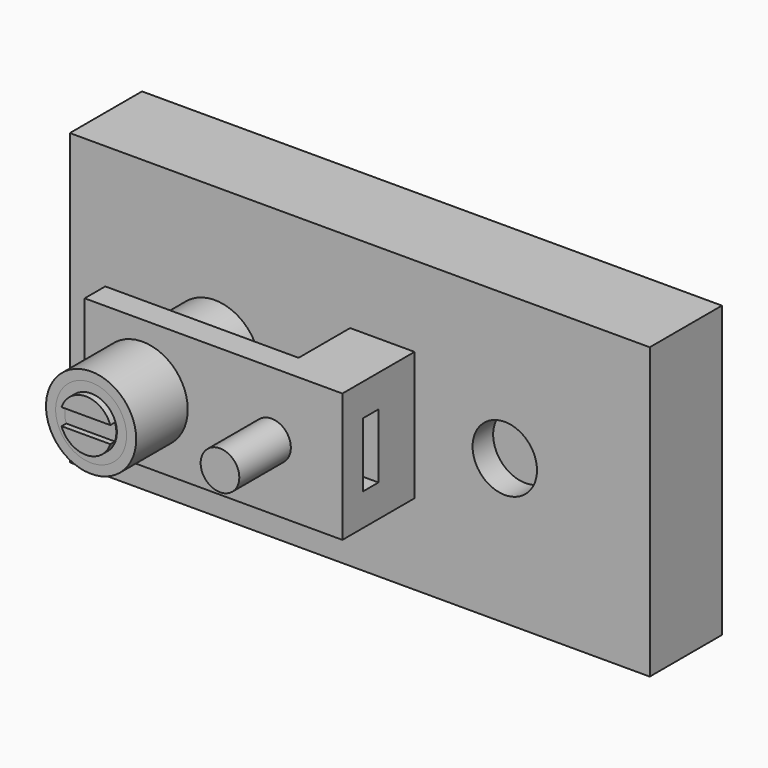
from build123d import *

# Parameters (mm, degrees)
F0_R           = 2.75
F1_DEPTH       = 7
F2_R           = 2
F3_DEPTH       = 9.9
F3_DEPTH_BACK  = 12.8
F4_R           = 3.5
F5_DEPTH       = 5
F6_R           = 2
F7_DEPTH       = 7.5
F9_START       = 7.05
F8_W           = 4
F8_H           = 1.3
F9_DEPTH       = 2
F10_W          = 20
F10_H          = 10
F11_DEPTH      = 2
F12_W          = 5
F12_H          = 5
F13_DEPTH      = 5
F14_W          = 1.5
F14_H          = 2.5
F15_DEPTH      = 22.67
F16_R          = 3.5
F16_R_2        = 2.75
F17_DEPTH      = 7
F18_R          = 2.75
F19_DEPTH      = 6.2
F19_DEPTH_BACK = 3.1
F23_START      = -5
F23_DEPTH      = 7
F25_START      = -7
F24_R          = 3.5
F25_DEPTH      = 7
F27_START      = -10
F26_W          = 32
F26_H          = 7
F27_DEPTH      = 15
F20_R          = 1.5
F28_DEPTH      = 7
F29_R          = 2.5
F30_DEPTH      = 10


with BuildPart() as f1:
    # F0 (on Front) → F1 (new body)
    with BuildSketch(Plane.XZ):
        Circle(F0_R)
    extrude(amount=F1_DEPTH)

    # F2 (on Front) → F3 (cut, two sides)
    with BuildSketch(Plane.XZ) as f3_sk:
        Circle(F2_R)
    extrude(amount=F3_DEPTH, mode=Mode.SUBTRACT)
    extrude(f3_sk.sketch, amount=-F3_DEPTH_BACK, mode=Mode.SUBTRACT)

    # F4 (on Front) → F5 (join)
    with BuildSketch(Plane.XZ):
        Circle(F4_R)
    extrude(amount=-F5_DEPTH)


with BuildPart() as f7:
    # F6 (on Front) → F7 (new body)
    with BuildSketch(Plane.XZ):
        Circle(F6_R)
    extrude(amount=F7_DEPTH)

    # F8 (on Front) → F9 (cut)
    with BuildSketch(Plane.XZ.offset(F9_START)):
        Rectangle(F8_W, F8_H)
    extrude(amount=F9_DEPTH, mode=Mode.SUBTRACT)


with BuildPart() as f11:
    # F10 (on Front) → F11 (new body)
    with BuildSketch(Plane.XZ):
        with Locations((5.5, 0)):
            Rectangle(F10_W, F10_H)
    extrude(amount=F11_DEPTH)

    # F12 (on Top) → F13 (join, symmetric)
    with BuildSketch(Plane.XY):
        with Locations((13, 2.5)):
            Rectangle(F12_W, F12_H)
    extrude(amount=F13_DEPTH, both=True)

    # F14 (on Right) → F15 (cut)
    with BuildSketch(Plane.YZ):
        with Locations((0.75, -1.25)):
            Rectangle(F14_W, F14_H)
        with Locations((0.75, 1.25)):
            Rectangle(F14_W, F14_H)
    extrude(amount=F15_DEPTH, mode=Mode.SUBTRACT)

    # F16 (on Front) → F17 (join)
    with BuildSketch(Plane.XZ):
        Circle(F16_R)
        Circle(F16_R_2, mode=Mode.SUBTRACT)
    extrude(amount=F17_DEPTH)

    # F18 (on Front) → F19 (cut, two sides)
    with BuildSketch(Plane.XZ) as f19_sk:
        Circle(F18_R)
    extrude(amount=F19_DEPTH, mode=Mode.SUBTRACT)
    extrude(f19_sk.sketch, amount=-F19_DEPTH_BACK, mode=Mode.SUBTRACT)

    # F20 (on Front) → F28 (join)
    with BuildSketch(Plane.XZ):
        with Locations((10, 0)):
            Circle(F20_R)
    extrude(amount=F28_DEPTH)


with BuildPart() as f23:
    # F22 (on Front) → F23 (new body)
    with BuildSketch(Plane.XZ.offset(F23_START)):
        Polygon((33.75, 11.25), (11.25, 11.25), (-11.25, 11.25), (-11.25, -11.25), (11.25, -11.25), (33.75, -11.25), align=None)
    extrude(amount=-F23_DEPTH)

    # F26 (on Front) → F27 (cut)
    with BuildSketch(Plane.XZ.offset(F27_START)):
        with Locations((11.1485, 0)):
            Rectangle(F26_W, F26_H)
    extrude(amount=-F27_DEPTH, mode=Mode.SUBTRACT)

    # F29 (on Front) → F30 (cut)
    with BuildSketch(Plane.XZ):
        with Locations((22.5, 0)):
            Circle(F29_R)
    extrude(amount=-F30_DEPTH, mode=Mode.SUBTRACT)


with BuildPart() as f25:
    # F24 (on Front) → F25 (new body)
    with BuildSketch(Plane.XZ.offset(F25_START)):
        Circle(F24_R)
    extrude(amount=-F25_DEPTH)


with BuildPart() as f25b:
    # F24 (on Front) → F25, piece 2 (new body)
    with BuildSketch(Plane.XZ.offset(F25_START)):
        with Locations((22.5, 0)):
            Circle(F24_R)
    extrude(amount=-F25_DEPTH)


solid = Compound([f1.part, f7.part, f11.part, f23.part, f25.part, f25b.part])
